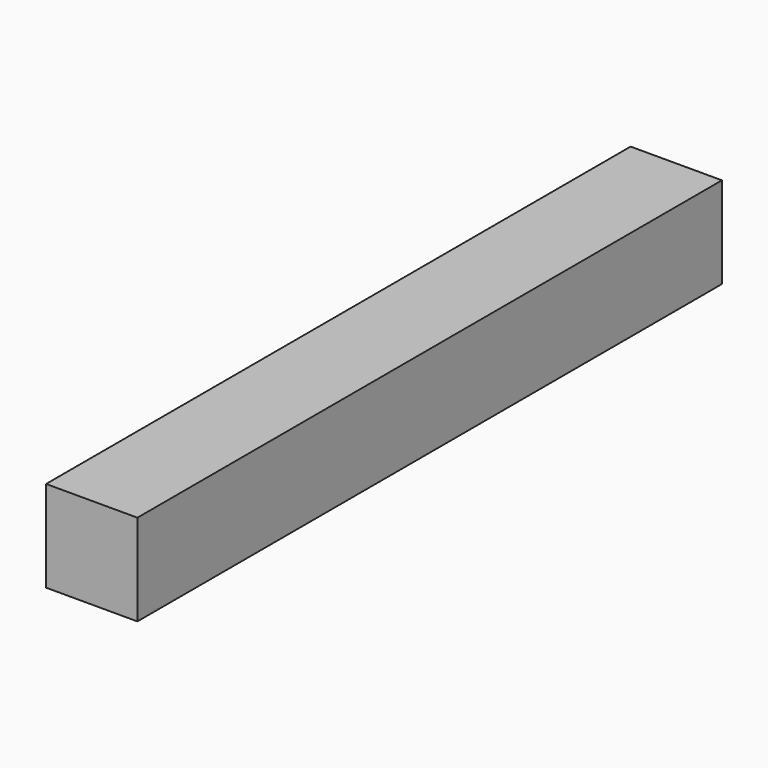
from build123d import *

# Parameters (mm, degrees)
F0_W     = 6
F0_H     = 6
F2_DEPTH = 48


with BuildPart() as f2:
    # F0 (on Front) → F2 (new body)
    with BuildSketch(Plane.XZ):
        with Locations((3, 3)):
            Rectangle(F0_W, F0_H)
    extrude(amount=F2_DEPTH)


solid = f2.part
